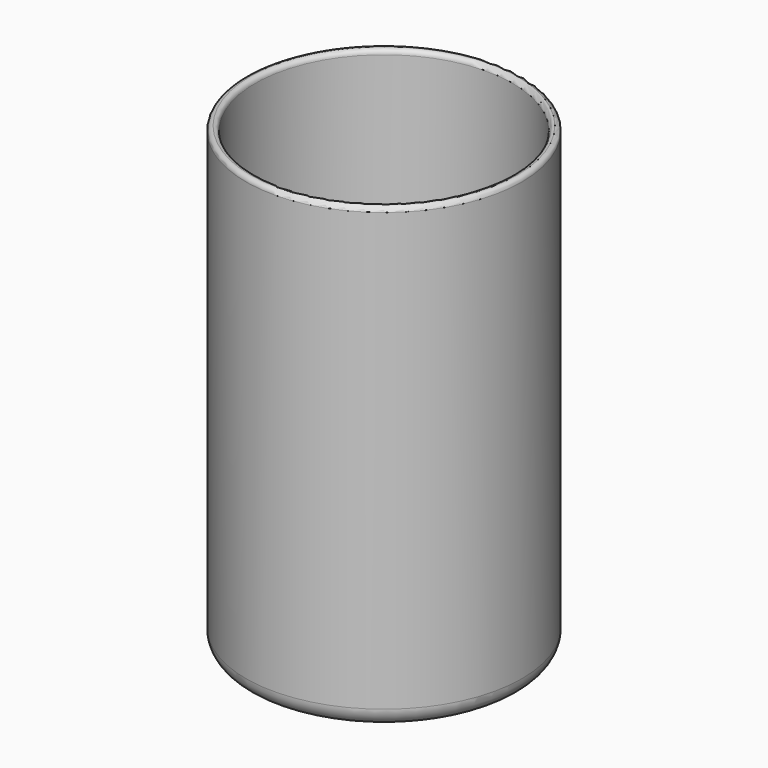
from build123d import *

# Parameters (mm, degrees)
F0_R     = 38.1
F0_R_2   = 35.56
F1_DEPTH = 127
F2_R     = 38.1
F3_DEPTH = 25.4
F4_R     = 1.26999
F5_R     = 5.08
F6_R     = 5.08


# Not quite as in the source:
# - a fillet or chamfer is up to 0.001 mm smaller than in the source, because OpenCascade refuses the exact size


with BuildPart() as f1:
    # F0 (on Top) → F1 (new body)
    with BuildSketch(Plane.XY):
        Circle(F0_R)
        Circle(F0_R_2, mode=Mode.SUBTRACT)
    extrude(amount=F1_DEPTH)

    # F2 (on Top) → F3 (join)
    with BuildSketch(Plane.XY):
        Circle(F2_R)
    extrude(amount=F3_DEPTH)

    # F4 (radius 1.27 in the source; OpenCascade refuses exactly that, so slightly less here)
    f4_edges = [f1.edges().sort_by_distance(p)[0] for p in [
        (-38.1, 0, 127),
        (-35.56, 0, 127),
    ]]
    fillet(f4_edges, radius=F4_R)

    # F5
    f5_edges = [f1.edges().sort_by_distance(p)[0] for p in [
        (-38.1, 0, 0),
    ]]
    fillet(f5_edges, radius=F5_R)

    # F6
    f6_edges = [f1.edges().sort_by_distance(p)[0] for p in [
        (-35.56, 0, 25.4),
    ]]
    fillet(f6_edges, radius=F6_R)


solid = f1.part
